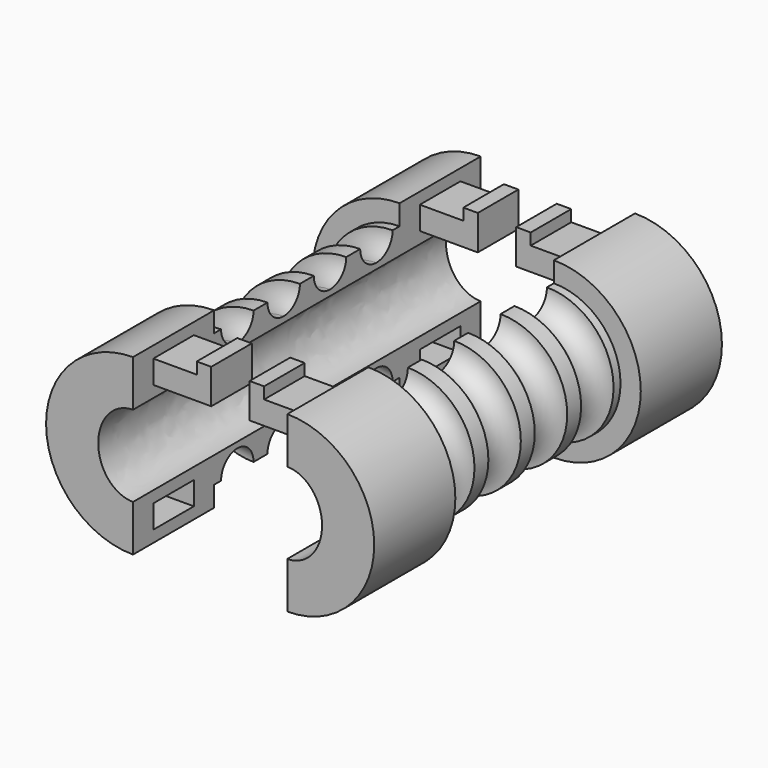
from build123d import *

# Parameters (mm, degrees)
F1_ANGLE_BACK = 90
F1_ANGLE      = 180
F3_DEPTH      = 190.5
F5_DEPTH      = 25.4
F7_DEPTH      = 25.4
F9_DEPTH      = 25.4
F11_DEPTH     = 25.4
F13_W         = 6.35
F13_H         = 22.225
F12_W         = 6.35
F12_H         = 22.225
F14_DEPTH     = 15.24


# Not quite as in the source:
# - a feature names something its author has since deleted; it is built from what else it names


with BuildPart() as f1:
    # F0 (on Top) → F1 (revolve)
    with BuildSketch(Plane.XY, mode=Mode.PRIVATE) as f1_sk:
        Polygon((-33.8094037018, 95.25), (-71.9094037018, 95.25), (-71.9094037018, 50.8), (-63.0194037018, 50.8), (-54.1294037018, 50.8), (-33.8094037018, 50.8), align=None)
        Polygon((-33.8094037018, -95.25), (-33.8094037018, 50.8), (-54.1294037018, 50.8), (-54.1294037018, 38.1), (-54.1294037018, 12.7000000718), (-54.1294037018, -12.6999999282), (-54.1294037018, -38.0999999341), (-54.1294037018, -50.8), (-63.0194037018, -50.8), (-71.9094037018, -50.8), (-71.9094037018, -95.25), align=None)
        with BuildLine():
            Line((-54.1294037018, 50.8), (-63.0194037018, 50.8))
            Line((-63.0194037018, 50.8), (-63.0194037018, 46.99))
            ThreePointArc((-63.0194037018, 46.99), (-56.733224417, 44.3861792847), (-54.1294037018, 38.1))
            Line((-54.1294037018, 38.1), (-54.1294037018, 50.8))
        make_face()
        with BuildLine():
            Line((-63.0194037018, -46.99), (-63.0194037018, -50.8))
            Line((-63.0194037018, -50.8), (-54.1294037018, -50.8))
            Line((-54.1294037018, -50.8), (-54.1294037018, -38.0999999341))
            ThreePointArc((-54.1294037018, -38.0999999341), (-56.7332243937, -44.3861792615), (-63.0194037018, -46.99))
        make_face()
        with BuildLine():
            Line((-54.1294037018, 12.7000000718), (-54.1294037018, 38.1))
            ThreePointArc((-54.1294037018, 38.1), (-56.733224417, 31.8138207153), (-63.0194037018, 29.21))
            Line((-63.0194037018, 29.21), (-63.0194037018, 21.59))
            ThreePointArc((-63.0194037018, 21.59), (-56.7332244424, 18.9861793101), (-54.1294037018, 12.7000000718))
        make_face()
        with BuildLine():
            Line((-54.1294037018, -12.6999999282), (-54.1294037018, 12.7000000718))
            ThreePointArc((-54.1294037018, 12.7000000718), (-56.7332243916, 6.4138207406), (-63.0194037018, 3.81))
            Line((-63.0194037018, 3.81), (-63.0194037018, 0))
            Line((-63.0194037018, 0), (-63.0194037018, -3.81))
            ThreePointArc((-63.0194037018, -3.81), (-56.7332244424, -6.4138206899), (-54.1294037018, -12.6999999282))
        make_face()
        with BuildLine():
            Line((-63.0194037018, -21.59), (-63.0194037018, -29.21))
            ThreePointArc((-63.0194037018, -29.21), (-56.7332244403, -31.813820692), (-54.1294037018, -38.0999999341))
            Line((-54.1294037018, -38.0999999341), (-54.1294037018, -12.6999999282))
            ThreePointArc((-54.1294037018, -12.6999999282), (-56.7332243916, -18.9861792594), (-63.0194037018, -21.59))
        make_face()
    revolve(f1_sk.sketch.rotate(Axis((-33.8094037018, 0, 0), (0, -1, 0)), -F1_ANGLE_BACK), axis=Axis((-33.8094037018, 0, 0), (0, -1, 0)), revolution_arc=F1_ANGLE)

    # F2 (on face) → F3 (cut)
    with BuildSketch(Plane.XZ.offset(95.25)):
        with BuildLine():
            add(Edge.make_bspline(
                [(-33.8094037018, 17.78), (-49.0494037018, 17.78), (-49.0494037018, 0)],
                knots=[3.1415926536, 3.1415926536, 3.1415926536, 4.7123889804, 4.7123889804, 4.7123889804], degree=2, weights=[1, 0.7071067812, 1]))
            add(Edge.make_bspline(
                [(-49.0494037018, 0), (-49.0494037018, -17.78), (-33.8094037018, -17.78)],
                knots=[4.7123889804, 4.7123889804, 4.7123889804, 6.2831853072, 6.2831853072, 6.2831853072], degree=2, weights=[1, 0.7071067812, 1]))
            Line((-33.8094037018, -17.78), (-33.8094037018, 17.78))
        make_face()
    extrude(amount=-F3_DEPTH, mode=Mode.SUBTRACT)

    # F4 (on face) → F5 (cut)
    with BuildSketch(Plane.YZ.offset(-33.8094037018)):
        Polygon((-84.1375, -22.86), (-84.1375, -27.94), (-84.1375, -33.02), (-61.9125, -33.02), (-61.9125, -22.86), align=None)
    extrude(amount=-F5_DEPTH, mode=Mode.SUBTRACT)

    # F6 (on face) → F7 (cut)
    with BuildSketch(Plane.YZ.offset(-33.8094037018)):
        Polygon((84.1375, -33.02), (84.1375, -27.94), (84.1375, -22.86), (61.9125, -22.86), (61.9125, -33.02), align=None)
    extrude(amount=-F7_DEPTH, mode=Mode.SUBTRACT)

    # F8 (on face) → F9 (join)
    with BuildSketch(Plane.YZ.offset(-33.8094037018)):
        Polygon((-84.1375, 33.02), (-84.1375, 27.94), (-84.1375, 22.86), (-61.9125, 22.86), (-61.9125, 33.02), align=None)
    extrude(amount=F9_DEPTH)

    # F10 (on face) → F11 (join)
    with BuildSketch(Plane.YZ.offset(-33.8094037018)):
        Polygon((84.1375, 22.86), (84.1375, 27.94), (84.1375, 33.02), (61.9125, 33.02), (61.9125, 22.86), align=None)
    extrude(amount=F11_DEPTH)

    # F13 (on face) + F12 (on face) → F14 (join)
    with BuildSketch(Plane(origin=(0, 0, 22.86), x_dir=(1, 0, 0), z_dir=(0, 0, -1))):
        with Locations((-11.5844037018, 73.025)):
            Rectangle(F13_W, F13_H)
    with BuildSketch(Plane(origin=(0, 0, 22.86), x_dir=(1, 0, 0), z_dir=(0, 0, -1))):
        with Locations((-11.5844037018, -73.025)):
            Rectangle(F12_W, F12_H)
    extrude(amount=-F14_DEPTH)


with BuildPart() as f15_1:
    # F15: instance of F1
    add(f1.part.mirror(Plane.YZ))


solid = Compound([f1.part, f15_1.part])
